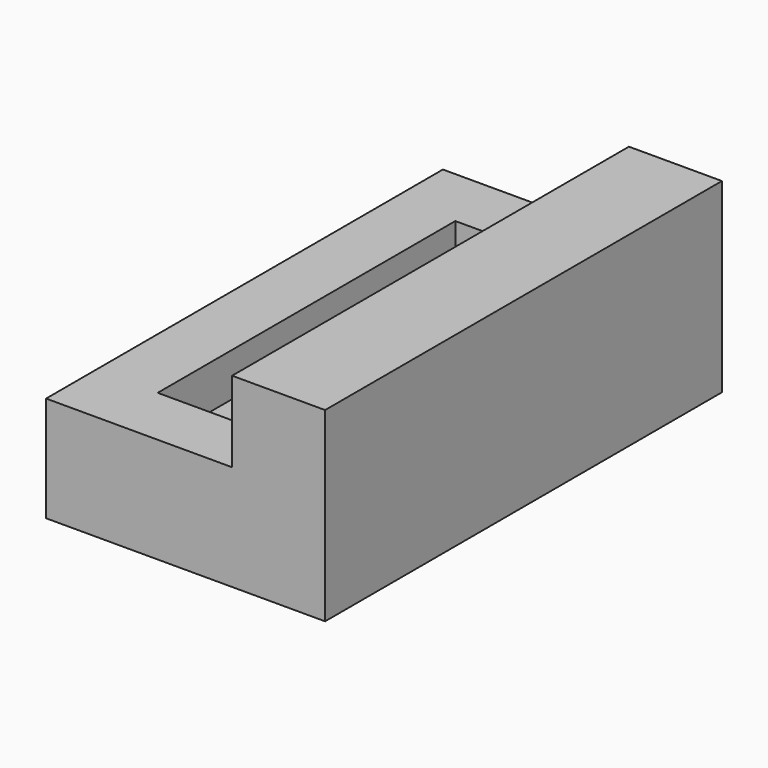
from build123d import *

# Parameters (mm, degrees)
F1_DEPTH      = 203.2
F2_W          = 25.4
F2_H          = 17.78
F3_DEPTH      = 50.8
F4_W          = 25.4
F4_H          = 17.78
F5_DEPTH      = 50.8
F11_DEPTH     = 0.0762
F31_T         = 2.54
F31_T3_DEPTH  = 30.48
F31_T5_DEPTH  = 22.86
F31_T7_DEPTH  = 157.48
F31_T9_DEPTH  = 30.48
F31_T11_DEPTH = 55.88


# Not quite as in the source:
# - a shell that OpenCascade refuses in one call is made with other operations: the cavity is built on its own and cut out
# - the program builds the solid bodies; features that only make, move or delete a surface that nothing else refers to are left out


with BuildPart() as f1:
    # F0 (on Front) → F1 (new body)
    with BuildSketch(Plane.XZ):
        Polygon((7.5239408249, -41.6093189047), (-17.8760591751, -41.6093189047), (-17.8760591751, -84.7893189047), (96.4239408249, -84.7893189047), (96.4239408249, -8.5893189047), (58.3239408249, -8.5893189047), (58.3239408249, -59.3893189047), (7.5239408249, -59.3893189047), align=None)
    extrude(amount=F1_DEPTH)

    # F2 (on face) → F3 (join)
    with BuildSketch(Plane.YZ.offset(7.5239408249)):
        with Locations((-190.5, -50.4993189047)):
            Rectangle(F2_W, F2_H)
    extrude(amount=F3_DEPTH)

    # F4 (on face) → F5 (join)
    with BuildSketch(Plane.YZ.offset(7.5239408249)):
        with Locations((-12.7, -50.4993189047)):
            Rectangle(F4_W, F4_H)
    extrude(amount=F5_DEPTH)

    # F9 (on face) → F11 (join)
    with BuildSketch(Plane(origin=(0, 0, 0), x_dir=(-1, 0, 0), z_dir=(0, 1, 0))):
        with BuildLine():
            ThreePointArc((-85.9858192503, -15.2795063332), (-92.0223010679, -14.3629027521), (-86.5299954351, -17.0300836035))
            ThreePointArc((-86.5299954351, -17.0300836035), (-86.12500001, -16.1961099143), (-85.9858192503, -15.2795063332))
        make_face()
    extrude(amount=F11_DEPTH)

    # F31: shell of thickness 2.54, made by hand


with BuildPart() as f31_core1:
    # F31_t2: copy of F1
    add(f1.part)

    # the walls: a layer under each face that stays
    f31_faces = [f31_core1.faces().sort_by_distance(p)[0] for p in [
        (77.3739408249, -101.6, -8.5893189047),
        (96.4239408249, -101.6, -46.6893189047),
        (58.3239408249, -101.6, -33.9893189047),
        (39.2739408249, 0, -46.6893189047),
        (39.2739408249, -203.2, -46.6893189047),
        (-5.1760591751, -33.8666666667, -41.6093189047),
        (32.9239408249, -25.4, -50.4993189047),
        (32.9239408249, -101.6, -59.3893189047),
        (32.9239408249, -177.8, -50.4993189047),
        (-17.8760591751, -101.6, -63.1993189047),
        (91.6173056428, 0.0381, -13.5289290629),
        (7.5239408249, -101.6, -50.4993189047),
        (89.0736505389, 0.0762, -15.2795063332),
    ]]
    thicken(f31_faces, amount=-F31_T, mode=Mode.SUBTRACT)

    # F31_s4 → F31_t3 (cut)
    with BuildSketch(Plane.XZ.offset(-2.54)):
        Polygon((58.2985408249, -41.5839189047), (60.8639408249, -41.6093189047), (60.8639408249, -44.1493189047), (58.3239408249, -44.1493189047), align=None)
    extrude(amount=F31_T3_DEPTH, mode=Mode.SUBTRACT)

    # F31_s6 → F31_t5 (cut)
    with BuildSketch(Plane.XY.offset(-61.9293189047)):
        Polygon((58.2985408249, -25.4254), (60.8639408249, -25.4), (60.8639408249, -22.86), (58.3239408249, -22.86), align=None)
        Polygon((58.2985408249, -177.7746), (60.8639408249, -177.8), (60.8639408249, -180.34), (58.3239408249, -180.34), align=None)
        Polygon((7.5493408249, -25.4254), (7.5239408249, -22.86), (4.9839408249, -22.86), (4.9839408249, -25.4), align=None)
        Polygon((7.5493408249, -177.7746), (7.5239408249, -180.34), (4.9839408249, -180.34), (4.9839408249, -177.8), align=None)
    extrude(amount=F31_T5_DEPTH, mode=Mode.SUBTRACT)

    # F31_s8 → F31_t7 (cut)
    with BuildSketch(Plane.XZ.offset(22.86)):
        Polygon((58.2985408249, -59.3639189047), (60.8639408249, -59.3893189047), (60.8639408249, -61.9293189047), (58.3239408249, -61.9293189047), align=None)
        Polygon((7.5493408249, -59.3639189047), (7.5239408249, -61.9293189047), (4.9839408249, -61.9293189047), (4.9839408249, -59.3893189047), align=None)
    extrude(amount=F31_T7_DEPTH, mode=Mode.SUBTRACT)

    # F31_s10 → F31_t9 (cut)
    with BuildSketch(Plane.XZ.offset(175.26)):
        Polygon((58.2985408249, -41.5839189047), (60.8639408249, -41.6093189047), (60.8639408249, -44.1493189047), (58.3239408249, -44.1493189047), align=None)
    extrude(amount=F31_T9_DEPTH, mode=Mode.SUBTRACT)

    # F31_s12 → F31_t11 (cut)
    with BuildSketch(Plane.YZ.offset(4.9839408249)):
        Polygon((-25.4254, -59.3639189047), (-22.86, -59.3893189047), (-22.86, -61.9293189047), (-25.4, -61.9293189047), align=None)
        Polygon((-177.7746, -59.3639189047), (-177.8, -61.9293189047), (-180.34, -61.9293189047), (-180.34, -59.3893189047), align=None)
    extrude(amount=F31_T11_DEPTH, mode=Mode.SUBTRACT)

    # F31_s13 → F31_t14 (revolve, cut)
    with BuildSketch(Plane(origin=(35.7646863661, 0, -51.9674444282), x_dir=(0, 1, 0), z_dir=(0.5669277583, 0, -0.8237675139))):
        Polygon((0.0254, 61.6003720947), (-2.54, 61.6257720947), (-2.54, 64.1657720947), (0, 64.1657720947), align=None)
    revolve(axis=Axis((89.0736505389, 0, -15.2795063332), (0, 1, 0)), mode=Mode.SUBTRACT)


with BuildPart() as f1_1:
    add(f1.part)

    # what is left inside the walls is the cavity
    f31_cavity = [f31_core1.part.solids().sort_by_distance(p)[0] for p in [
        (39.273941, -134.62, -84.763919),
    ]]
    add(f31_cavity, mode=Mode.SUBTRACT)


solid = f1_1.part
